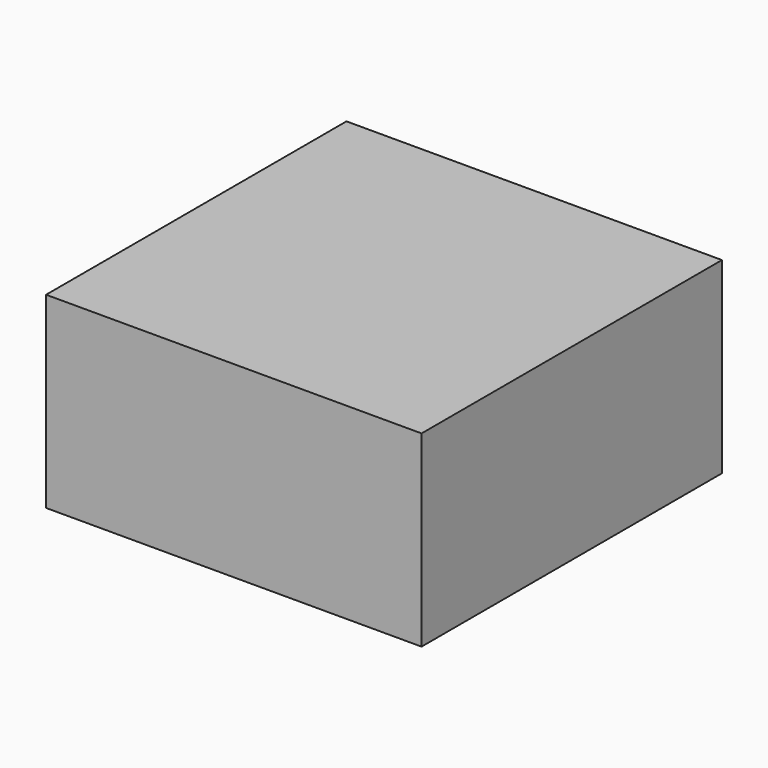
from build123d import *

# Parameters (mm, degrees)
F0_W     = 12
F0_H     = 12
F1_DEPTH = 6


# Not quite as in the source:
# - the program builds the solid bodies; features that only make, move or delete a surface that nothing else refers to are left out


with BuildPart() as f1:
    # F0 (on Top) → F1 (new body)
    with BuildSketch(Plane.XY):
        Rectangle(F0_W, F0_H)
    extrude(amount=F1_DEPTH)


solid = f1.part
